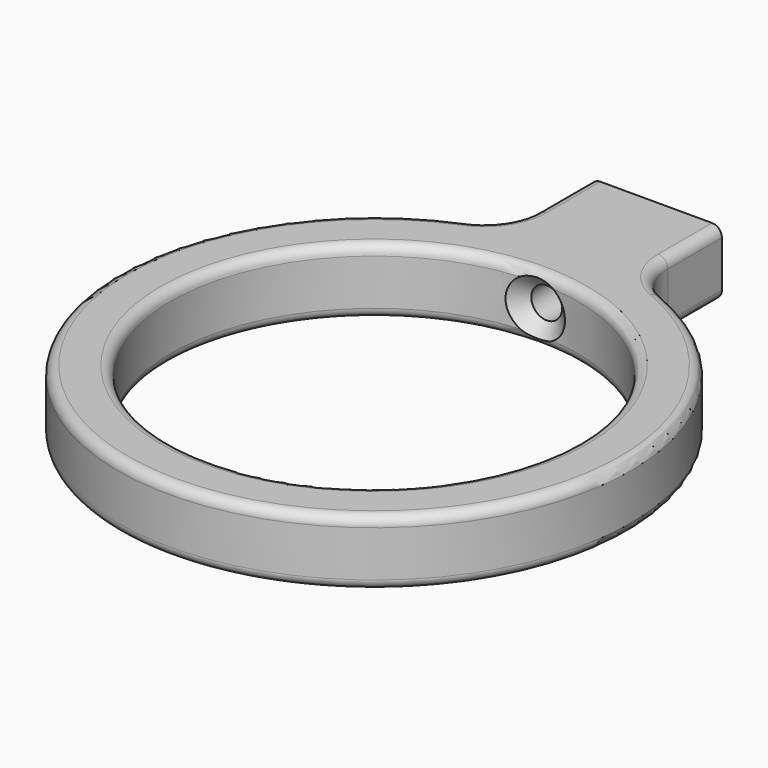
from build123d import *

# Parameters (mm, degrees)
F0_R         = 31
F1_DEPTH     = 10
F2_R         = 2.35
F3_DEPTH     = 22.7863546661
F6_T1_DEPTH  = 14.0295669578
F6_T4_ANGLE  = 314.9633717383
F6_T6_ANGLE  = 314.9633717383
F6_T12_ANGLE = 67.4816858691
F6_T14_ANGLE = 67.4816858691
F6_T16_ANGLE = 67.4816858691
F6_T18_ANGLE = 67.4816858691


# Not quite as in the source:
# - a fillet or chamfer that OpenCascade refuses, or shapes differently, is made with other operations: its cross-section is extruded or revolved along the edge and cut away or added


with BuildPart() as f1:
    # F0 (on Top) → F1 (new body)
    with BuildSketch(Plane.XY):
        with BuildLine():
            ThreePointArc((-10, 43.4165866922), (-11.3475328525, 38.9730879748), (-14.9361702128, 36.0265293829))
            ThreePointArc((-14.9361702128, 36.0265293829), (0, -39), (14.9361702128, 36.0265293829))
            ThreePointArc((14.9361702128, 36.0265293829), (11.3475328525, 38.9730879748), (10, 43.4165866922))
            Line((10, 43.4165866922), (10, 53.6961536499))
            Line((10, 53.6961536499), (-10, 53.6961536499))
            Line((-10, 53.6961536499), (-10, 43.4165866922))
        make_face()
        Circle(F0_R, mode=Mode.SUBTRACT)
    extrude(amount=F1_DEPTH)

    # F2 (on face) → F3 (cut, through all)
    with BuildSketch(Plane(origin=(0, 53.6961536499, 0), x_dir=(-1, 0, 0), z_dir=(0, 1, 0))):
        with Locations((0, 5)):
            Circle(F2_R)
    extrude(amount=-F3_DEPTH, mode=Mode.SUBTRACT)

    # F4 (on Right) → F5 (revolve, cut)
    with BuildSketch(Plane.YZ):
        Polygon((35.1961536499, 5), (30.1961536499, 10), (30.1961536499, 5), align=None)
    revolve(axis=Axis((0, 32.6961536499, 5), (0, -1, 0)), mode=Mode.SUBTRACT)

    # F6: fillet of radius 1.5 on 12 edges, made by hand

    # F6_s2 → F6_t1 (cut)
    with BuildSketch(Plane.XZ.offset(-57.4461536499)):
        with BuildLine():
            ThreePointArc((-10, 1.5), (-9.5606601718, 0.4393398282), (-8.5, 0))
            Line((-8.5, 0), (-10, 0))
            Line((-10, 0), (-10, 1.5))
        make_face()
        with BuildLine():
            ThreePointArc((-10, 8.5), (-9.5606601718, 9.5606601718), (-8.5, 10))
            Line((-8.5, 10), (-10, 10))
            Line((-10, 10), (-10, 8.5))
        make_face()
        with BuildLine():
            ThreePointArc((8.5, 0), (9.5606601718, 0.4393398282), (10, 1.5))
            Line((10, 1.5), (10, 0))
            Line((10, 0), (8.5, 0))
        make_face()
        with BuildLine():
            ThreePointArc((8.5, 10), (9.5606601718, 9.5606601718), (10, 8.5))
            Line((10, 8.5), (10, 10))
            Line((10, 10), (8.5, 10))
        make_face()
    extrude(amount=F6_T1_DEPTH, mode=Mode.SUBTRACT)

    # F6_s3 → F6_t4 (revolve, cut)
    with BuildSketch(Plane(origin=(0, 0, 0), x_dir=(0, 0, 1), z_dir=(0.9237571637, 0.3829787234, 0))):
        with BuildLine():
            ThreePointArc((8.5, -39), (9.5606601718, -38.5606601718), (10, -37.5))
            Line((10, -37.5), (10, -39))
            Line((10, -39), (8.5, -39))
        make_face()
    revolve(axis=Axis((0, 0, 10), (0, 0, 1)), revolution_arc=F6_T4_ANGLE, mode=Mode.SUBTRACT)

    # F6_s5 → F6_t6 (revolve, cut)
    with BuildSketch(Plane(origin=(0, 0, 0), x_dir=(0, 0, 1), z_dir=(0.9237571637, 0.3829787234, 0))):
        with BuildLine():
            ThreePointArc((1.5, -39), (0.4393398282, -38.5606601718), (0, -37.5))
            Line((0, -37.5), (0, -39))
            Line((0, -39), (1.5, -39))
        make_face()
    revolve(axis=Axis((0, 0, 0), (0, 0, 1)), revolution_arc=F6_T6_ANGLE, mode=Mode.SUBTRACT)

    # F6_s7 → F6_t8 (revolve, cut)
    with BuildSketch(Plane.XZ):
        with BuildLine():
            ThreePointArc((32.5, 0), (31.4393398282, 0.4393398282), (31, 1.5))
            Line((31, 1.5), (31, 0))
            Line((31, 0), (32.5, 0))
        make_face()
    revolve(axis=Axis((0, 0, 0), (0, 0, 1)), mode=Mode.SUBTRACT)

    # F6_s9 → F6_t10 (revolve, cut)
    with BuildSketch(Plane.XZ):
        with BuildLine():
            ThreePointArc((32.5, 10), (31.4393398282, 9.5606601718), (31, 8.5))
            Line((31, 8.5), (31, 10))
            Line((31, 10), (32.5, 10))
        make_face()
    revolve(axis=Axis((0, 0, 10), (0, 0, 1)), mode=Mode.SUBTRACT)

    # F6_s11 → F6_t12 (revolve, cut)
    with BuildSketch(Plane.XZ.offset(-43.4165866922)):
        with BuildLine():
            ThreePointArc((-10, 1.5), (-9.5606601718, 0.4393398282), (-8.5, 0))
            Line((-8.5, 0), (-10, 0))
            Line((-10, 0), (-10, 1.5))
        make_face()
    revolve(axis=Axis((-18, 43.4165866922, 0), (0, 0, -1)), revolution_arc=F6_T12_ANGLE, mode=Mode.SUBTRACT)

    # F6_s13 → F6_t14 (revolve, cut)
    with BuildSketch(Plane.XZ.offset(-43.4165866922)):
        with BuildLine():
            ThreePointArc((-10, 8.5), (-9.5606601718, 9.5606601718), (-8.5, 10))
            Line((-8.5, 10), (-10, 10))
            Line((-10, 10), (-10, 8.5))
        make_face()
    revolve(axis=Axis((-18, 43.4165866922, 10), (0, 0, -1)), revolution_arc=F6_T14_ANGLE, mode=Mode.SUBTRACT)

    # F6_s15 → F6_t16 (revolve, cut)
    with BuildSketch(Plane(origin=(0, 0, 0), x_dir=(0, 0, 1), z_dir=(0.9237571637, -0.3829787234, 0))):
        with BuildLine():
            ThreePointArc((0, -37.5), (0.4393398282, -38.5606601718), (1.5, -39))
            Line((1.5, -39), (0, -39))
            Line((0, -39), (0, -37.5))
        make_face()
    revolve(axis=Axis((18, 43.4165866922, 0), (0, 0, -1)), revolution_arc=F6_T16_ANGLE, mode=Mode.SUBTRACT)

    # F6_s17 → F6_t18 (revolve, cut)
    with BuildSketch(Plane(origin=(0, 0, 0), x_dir=(0, 0, 1), z_dir=(0.9237571637, -0.3829787234, 0))):
        with BuildLine():
            ThreePointArc((10, -37.5), (9.5606601718, -38.5606601718), (8.5, -39))
            Line((8.5, -39), (10, -39))
            Line((10, -39), (10, -37.5))
        make_face()
    revolve(axis=Axis((18, 43.4165866922, 10), (0, 0, -1)), revolution_arc=F6_T18_ANGLE, mode=Mode.SUBTRACT)


solid = f1.part
